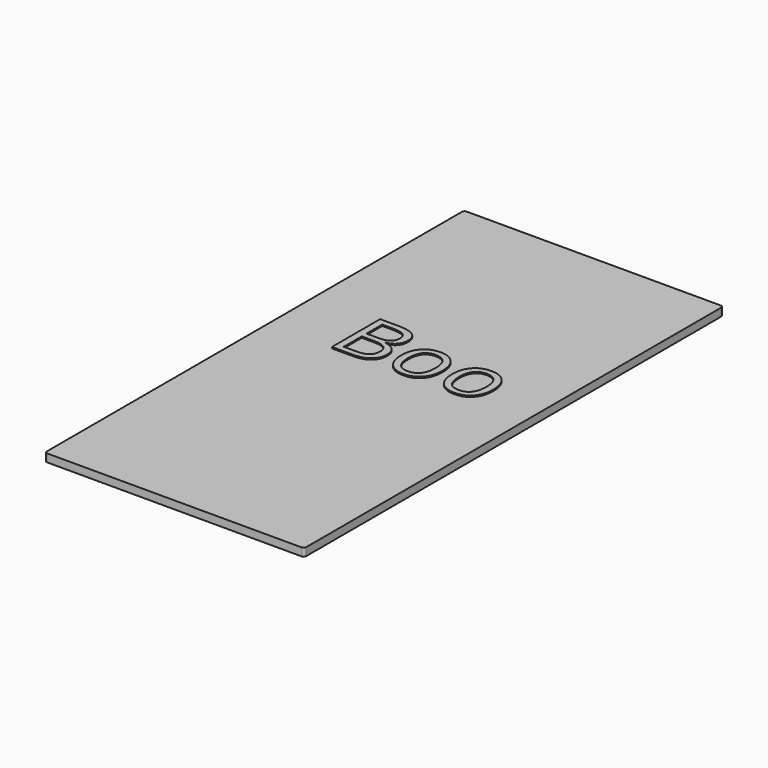
from build123d import *

# Parameters (mm, degrees)
F0_W         = 98
F0_H         = 198
F1_DEPTH     = 3
F2_R         = 0.9
F3_R         = 1
F4_TEXT_SIZE = 32.7316837178
F5_DEPTH     = 1
F6_TEXT_SIZE = 31.8578547902
F7_DEPTH     = 3.5


# Not quite as in the source:
# - Text() gives the source's letters only with a copy of the font that has no kerning and outlines rounded to 1/6400 em; it was checked with that copy


with BuildPart() as f1:
    # F0 (on Top) → F1 (new body)
    with BuildSketch(Plane.XY):
        with Locations((49, 99)):
            Rectangle(F0_W, F0_H)
    extrude(amount=F1_DEPTH)

    # F2
    f2_edges = [f1.edges().sort_by_distance(p)[0] for p in [
        (0, 0, 1.5),
        (98, 0, 1.5),
    ]]
    fillet(f2_edges, radius=F2_R)

    # F3
    f3_edges = [f1.edges().sort_by_distance(p)[0] for p in [
        (0, 198, 1.5),
        (98, 198, 1.5),
    ]]
    fillet(f3_edges, radius=F3_R)

    # F4 (on face) → F5 (join)
    with BuildSketch(Plane.XY.offset(3)):
        with Locations((13.076451607, 103.1266748905)):
            Text('Boo!', F4_TEXT_SIZE, font='Open Sans', text_align=(TextAlign.LEFT, TextAlign.BOTTOM))
    extrude(amount=-F5_DEPTH)

    # F6 (on Top) → F7 (join)
    with BuildSketch(Plane.XY):
        with Locations((21.4757844806, 104.8783659935)):
            Text('Boo', F6_TEXT_SIZE, font='Open Sans', text_align=(TextAlign.LEFT, TextAlign.BOTTOM))
    extrude(amount=F7_DEPTH)


solid = f1.part
